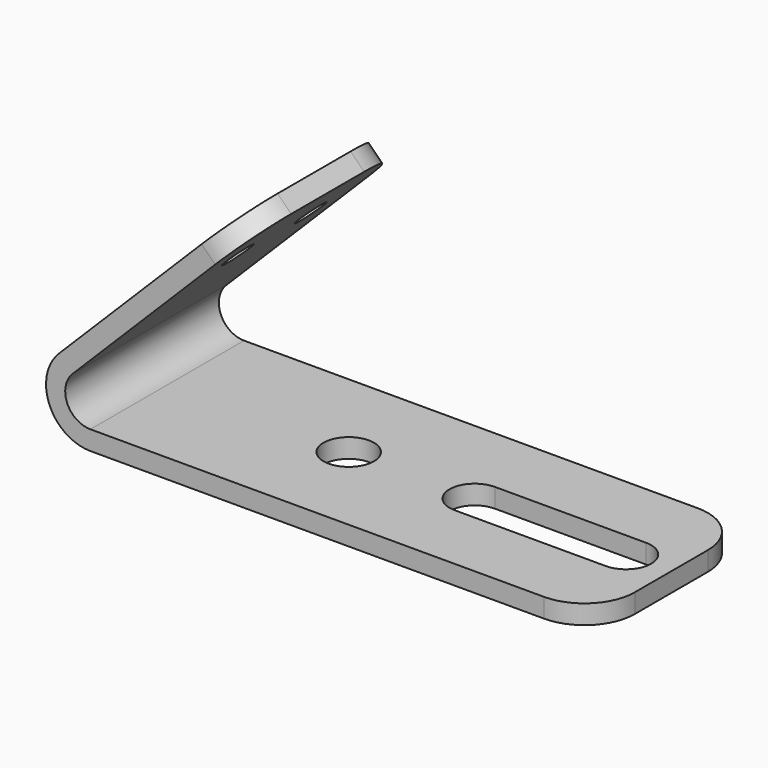
from build123d import *

# Parameters (mm, degrees)
F1_DEPTH = 241.935
F2_R     = 63.5
F3_DEPTH = 48.261
F4_R     = 38.1
F5_DEPTH = 48.26
F6_R     = 127
F7_R     = 127


# Not quite as in the source:
# - a pattern or mirror of a feature is missing from the dataset's text; its kind, count and spacing are read off the source's solid


with BuildPart() as f1:
    # F0 (on Front) → F1 (new body, symmetric)
    with BuildSketch(Plane.XZ):
        with BuildLine():
            Line((-1270, 0), (0, 0))
            Line((0, 0), (0, 48.26))
            Line((0, 48.26), (-1270, 48.26))
            ThreePointArc((-1270, 48.26), (-1328.6663503145, 87.4596020448), (-1314.9012806053, 156.6612806053))
            Line((-1314.9012806053, 156.6612806053), (-865.8884745519, 605.6740866588))
            Line((-865.8884745519, 605.6740866588), (-900.013447812, 639.7990599189))
            Line((-900.013447812, 639.7990599189), (-1349.0262538654, 190.7862538654))
            ThreePointArc((-1349.0262538654, 190.7862538654), (-1373.2527765535, 68.9912995989), (-1270, 0))
        make_face()
    extrude(amount=F1_DEPTH, both=True)

    # F2 (on face) → F3 (cut, through all)
    with BuildSketch(Plane.XY.offset(48.26)):
        with Locations((-812.8, 0)):
            Circle(F2_R)
        with BuildLine():
            ThreePointArc((-495.3, -63.5), (-450.3987193947, -44.9012806053), (-431.8, 0))
            ThreePointArc((-431.8, 0), (-450.3987193947, 44.9012806053), (-495.3, 63.5))
            ThreePointArc((-495.3, 63.5), (-558.8, 0), (-495.3, -63.5))
        make_face()
        with BuildLine():
            ThreePointArc((-495.3, 63.5), (-450.3987193947, 44.9012806053), (-431.8, 0))
            ThreePointArc((-431.8, 0), (-450.3987193947, -44.9012806053), (-495.3, -63.5))
            Line((-495.3, -63.5), (-114.3, -63.5))
            ThreePointArc((-114.3, -63.5), (-177.8, 0), (-114.3, 63.5))
            Line((-114.3, 63.5), (-495.3, 63.5))
        make_face()
        with BuildLine():
            ThreePointArc((-50.8, 0), (-69.3987193947, 44.9012806053), (-114.3, 63.5))
            ThreePointArc((-114.3, 63.5), (-177.8, 0), (-114.3, -63.5))
            ThreePointArc((-114.3, -63.5), (-69.3987193947, -44.9012806053), (-50.8, 0))
        make_face()
    extrude(amount=-F3_DEPTH, mode=Mode.SUBTRACT)

    # F4 (on face) → F5 (cut, through all)
    with BuildSketch(Plane(origin=(-769.9062538654, 0, 769.9062538654), x_dir=(0, -1, 0), z_dir=(-0.7071067812, 0, 0.7071067812))):
        with Locations((114.3, -374.4993582415)):
            Circle(F4_R)
    f5 = extrude(amount=-F5_DEPTH, mode=Mode.SUBTRACT)

    # F5_copies: F5 across plane
    add(f5.mirror(Plane.ZX), mode=Mode.SUBTRACT)

    # F6
    f6_edges = [f1.edges().sort_by_distance(p)[0] for p in [
        (-882.950961, 241.935, 622.736573),
        (-882.950961, -241.935, 622.736573),
    ]]
    fillet(f6_edges, radius=F6_R)

    # F7
    f7_edges = [f1.edges().sort_by_distance(p)[0] for p in [
        (0, 241.935, 24.13),
        (0, -241.935, 24.13),
    ]]
    fillet(f7_edges, radius=F7_R)


solid = f1.part
